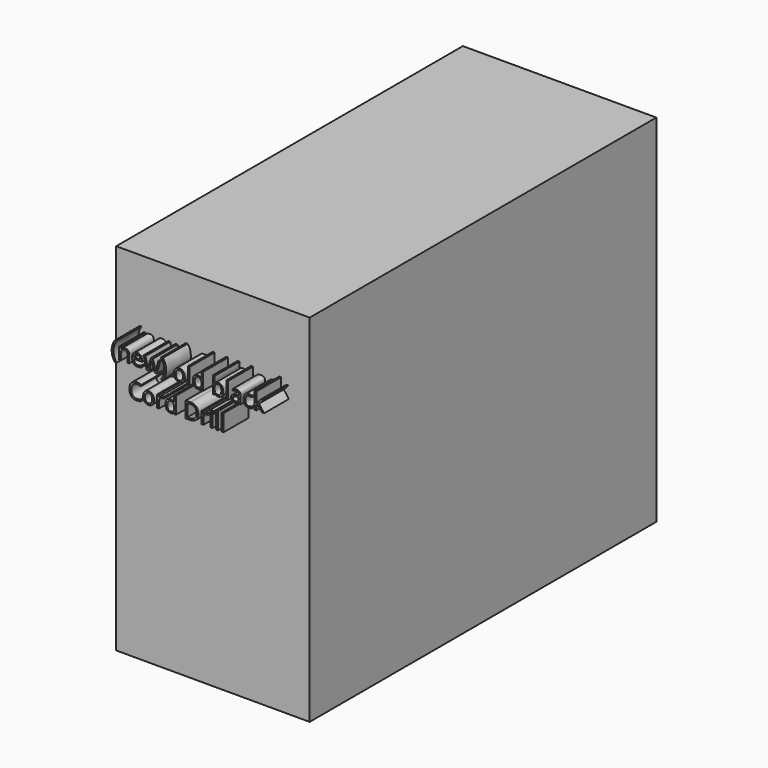
from build123d import *

# Parameters (mm, degrees)
F0_W         = 158.75
F0_H         = 292.1
F1_DEPTH     = 355.6
F2_TEXT_SIZE = 18.1141494506
F3_DEPTH     = 25.4


# Not quite as in the source:
# - Text() gives the source's letters only with a copy of the font that has no kerning and outlines rounded to 1/6400 em; it was checked with that copy


with BuildPart() as f1:
    # F0 (on Front) → F1 (new body)
    with BuildSketch(Plane.XZ):
        Rectangle(F0_W, F0_H)
    extrude(amount=F1_DEPTH)

    # F2 (on face) → F3 (join)
    with BuildSketch(Plane.XZ.offset(355.6)):
        with Locations((-63.5, 81.7072949573)):
            Text('(new) old black', F2_TEXT_SIZE, font='Open Sans', text_align=(TextAlign.LEFT, TextAlign.BOTTOM))
        with Locations((-49.379454436, 57.0720517044)):
            Text('Cord Drill', F2_TEXT_SIZE, font='Open Sans', text_align=(TextAlign.LEFT, TextAlign.BOTTOM))
    extrude(amount=F3_DEPTH)


solid = f1.part
